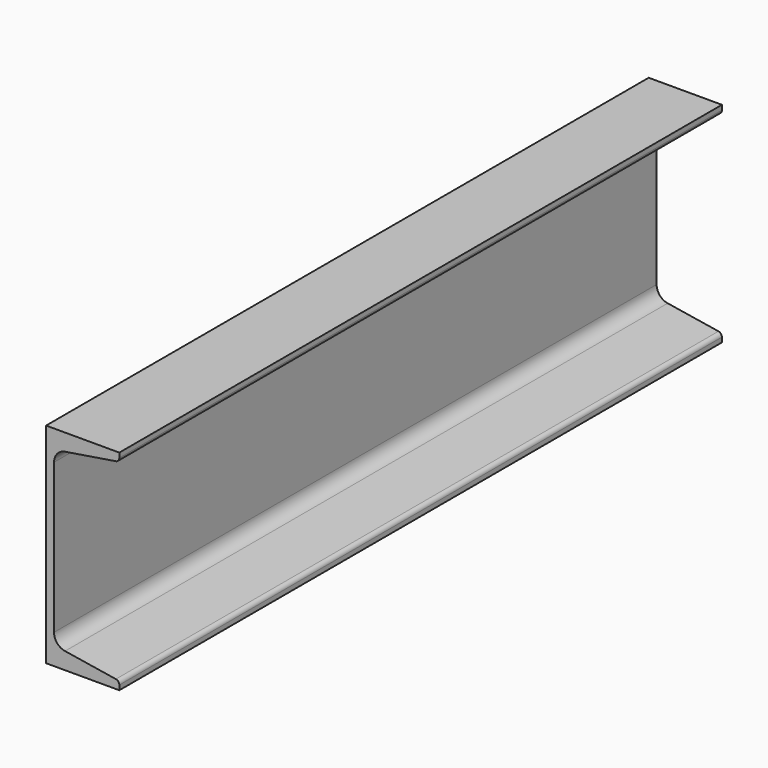
from build123d import *

# Parameters (mm, degrees)
F1_DEPTH = 457.2
F0_W     = 25.4
F0_H     = 49.170082
F0_H_2   = 8.8030812
F0_H_3   = 4.7118778
F0_W_2   = 31.496
F0_H_4   = 25.4
F0_W_3   = 6.5532254
F0_H_5   = 4.729226
F0_H_6   = 8.769477
F0_H_7   = 49.202594
F0_W_4   = 31.3436
F0_W_5   = 9.0424
F0_H_8   = 4.724908
F0_H_9   = 8.777859
F0_H_10  = 49.194466
F0_H_11  = 4.9884076
F0_H_12  = 10.7895644
F0_H_13  = 70.044056
F0_W_6   = 35.56
F0_W_7   = 8.1534
F0_H_14  = 90.86723
F0_H_15  = 12.7743204
F0_H_16  = 5.2920646
F0_W_8   = 39.6239238
F0_W_9   = 8.2550254
F0_H_17  = 7.9246984
F0_H_18  = 11.1253016
F0_H_19  = 88.9
F0_H_20  = 11.1252762
F0_H_21  = 7.9247238
F0_H_22  = 7.9249016
F0_H_23  = 12.7
F0_H_24  = 111.1501968
F0_W_10  = 46.8120476
F0_W_11  = 7.9756762
F0_H_25  = 111.1505778
F0_W_12  = 55.5499016
F0_W_13  = 7.8739238
F0_H_26  = 11.0997238
F0_H_27  = 9.525
F0_H_28  = 11.0996984
F0_H_29  = 111.1503746
F0_W_14  = 43.6878222
F0_W_15  = 11.0999016
F0_W_16  = 66.675
F0_W_17  = 8.0264508
F0_H_30  = 14.2746984
F0_H_31  = 98.4505778
F0_H_32  = 14.2747238
F0_W_18  = 80.2641016
F0_W_19  = 8.6358984
F0_H_33  = 20.6247238
F0_H_34  = 6.35
F0_H_35  = 20.6246984


# Not quite as in the source:
# - ends of sketch curves that miss each other by under 0.0002 mm in the source are joined


with BuildPart() as f1:
    # F0 (on Front) → F1 (new body)
    with BuildSketch(Plane.XZ):
        with BuildLine():
            Line((-601.1868342, 387.2012576), (-601.1868342, 311.0012576))
            Line((-601.1868342, 311.0012576), (-565.3728342, 311.0012576))
            Line((-565.3728342, 311.0012576), (-565.3728342, 313.5336122))
            ThreePointArc((-565.3728342, 313.5336122), (-565.9005539947, 314.9657928472), (-567.2313750211, 315.7131515187))
            Line((-567.2313750211, 315.7131515187), (-592.8587584, 319.8135336))
            ThreePointArc((-592.8587584, 319.8135336), (-595.7302015679, 321.4260723396), (-596.8688342, 324.5162166))
            Line((-596.8688342, 324.5162166), (-596.8688342, 373.6862986))
            ThreePointArc((-596.8688342, 373.6862986), (-595.7302015679, 376.7764428604), (-592.8587590083, 378.388985402))
            Line((-592.8587590083, 378.388985402), (-567.2313776, 382.4893798))
            ThreePointArc((-567.2313776, 382.4893798), (-565.9005539947, 383.2367223528), (-565.3728342, 384.668903))
            Line((-565.3728342, 384.668903), (-565.3728342, 387.2012576))
            Line((-565.3728342, 387.2012576), (-601.1868342, 387.2012576))
        make_face()
    extrude(amount=F1_DEPTH)


with BuildPart() as f1b:
    # F0 (on Front) → F1, piece 2 (new body)
    with BuildSketch(Plane.XZ):
        Polygon((-490.1583542, 311.0012576), (-458.6623542, 311.0012576), (-458.6623542, 336.4012576), (-490.1583542, 336.4012576), (-490.1583542, 315.3192576), align=None)
        Polygon((-494.4763542, 311.0012576), (-490.1583542, 311.0012576), (-490.1583542, 315.3192576), align=None)
        Polygon((-490.1583542, 315.3192576), (-490.1583542, 336.4012576), (-494.4763542, 336.4012576), (-494.4763542, 311.0012576), align=None)
    extrude(amount=F1_DEPTH)


with BuildPart() as f1c:
    # F0 (on Front) → F1, piece 3 (new body)
    with BuildSketch(Plane.XZ):
        with Locations((-369.8588742, 349.1012576)):
            Rectangle(F0_W, F0_H)
        with Locations((-369.8588742, 378.0878392)):
            Rectangle(F0_W, F0_H_2)
        with Locations((-369.8588742, 384.8453187)):
            Rectangle(F0_W, F0_H_3)
        Polygon((-357.1588742, 315.7131354), (-357.1588742, 324.5162166), (-382.5588742, 324.5162166), (-382.5588742, 315.7131354), (-377.8469964, 315.7131354), align=None)
        Polygon((-357.1588742, 311.0012576), (-357.1588742, 315.7131354), (-377.8469964, 315.7131354), (-382.5588742, 311.0012576), align=None)
        Polygon((-377.8469964, 315.7131354), (-382.5588742, 315.7131354), (-382.5588742, 311.0012576), align=None)
    extrude(amount=F1_DEPTH)


with BuildPart() as f1d:
    # F0 (on Front) → F1, piece 4 (new body)
    with BuildSketch(Plane.XZ):
        with BuildLine():
            Line((-282.0713942, 387.2012576), (-282.0713942, 311.0012576))
            Line((-282.0713942, 311.0012576), (-244.2253942, 311.0012576))
            Line((-244.2253942, 311.0012576), (-244.2253942, 313.542934))
            ThreePointArc((-244.2253942, 313.542934), (-244.755053678, 314.9803842916), (-246.0907679772, 315.7304974926))
            Line((-246.0907679772, 315.7304974926), (-271.5081184, 319.7972776))
            ThreePointArc((-271.5081184, 319.7972776), (-274.3795615679, 321.4098163396), (-275.5181942, 324.4999606))
            Line((-275.5181942, 324.4999606), (-275.5181942, 373.7025546))
            ThreePointArc((-275.5181942, 373.7025546), (-274.3795615679, 376.7926988604), (-271.5081190083, 378.405241402))
            Line((-271.5081190083, 378.405241402), (-246.0907702, 382.4720316))
            ThreePointArc((-246.0907702, 382.4720316), (-244.755053678, 383.2221309084), (-244.2253942, 384.6595812))
            Line((-244.2253942, 384.6595812), (-244.2253942, 387.2012576))
            Line((-244.2253942, 387.2012576), (-282.0713942, 387.2012576))
        make_face()
    extrude(amount=F1_DEPTH)


with BuildPart() as f1e:
    # F0 (on Front) → F1, piece 5 (new body)
    with BuildSketch(Plane.XZ):
        with Locations((-153.1612888, 323.7012576)):
            Rectangle(F0_W_2, F0_H_4)
        with Locations((-172.1859015, 323.7012576)):
            Rectangle(F0_W_3, F0_H_4)
    extrude(amount=F1_DEPTH)


with BuildPart() as f1f:
    # F0 (on Front) → F1, piece 6 (new body)
    with BuildSketch(Plane.XZ):
        with Locations((-49.7274342, 384.8366446)):
            Rectangle(F0_W, F0_H_5)
        with Locations((-49.7274342, 378.0872931)):
            Rectangle(F0_W, F0_H_6)
        with Locations((-49.7274342, 349.1012576)):
            Rectangle(F0_W, F0_H_7)
        Polygon((-37.0274342, 324.4999606), (-62.4274342, 324.4999606), (-62.4274342, 315.7304836), (-57.6982082, 315.7304836), (-37.0274342, 315.7304836), align=None)
        Polygon((-57.6982082, 315.7304836), (-62.4274342, 315.7304836), (-62.4274342, 311.0012576), align=None)
        Polygon((-57.6982082, 315.7304836), (-62.4274342, 311.0012576), (-37.0274342, 311.0012576), (-37.0274342, 315.7304836), align=None)
    extrude(amount=F1_DEPTH)


with BuildPart() as f1g:
    # F0 (on Front) → F1, piece 7 (new body)
    with BuildSketch(Plane.XZ):
        with BuildLine():
            Line((36.7900458, 387.2012576), (36.7900458, 311.0012576))
            Line((36.7900458, 311.0012576), (77.1760458, 311.0012576))
            Line((77.1760458, 311.0012576), (77.1760458, 313.5405972))
            ThreePointArc((77.1760458, 313.5405972), (76.6468679067, 314.9767339928), (75.3123701078, 315.7261562738))
            Line((75.3123701078, 315.7261562738), (49.8425216, 319.8013416))
            ThreePointArc((49.8425216, 319.8013416), (46.9710784321, 321.4138803396), (45.8324458, 324.5040246))
            Line((45.8324458, 324.5040246), (45.8324458, 373.6984906))
            ThreePointArc((45.8324458, 373.6984906), (46.9710784321, 376.7886348604), (49.8425209917, 378.401177402))
            Line((49.8425209917, 378.401177402), (75.3123716, 382.4763496))
            ThreePointArc((75.3123716, 382.4763496), (76.6468679067, 383.2257812072), (77.1760458, 384.661918))
            Line((77.1760458, 384.661918), (77.1760458, 387.2012576))
            Line((77.1760458, 387.2012576), (36.7900458, 387.2012576))
        make_face()
    extrude(amount=F1_DEPTH)


with BuildPart() as f1h:
    # F0 (on Front) → F1, piece 8 (new body)
    with BuildSketch(Plane.XZ):
        with Locations((168.2020258, 323.7012576)):
            Rectangle(F0_W_4, F0_H_4)
        with Locations((148.0090258, 323.7012576)):
            Rectangle(F0_W_5, F0_H_4)
    extrude(amount=F1_DEPTH)


with BuildPart() as f1i:
    # F0 (on Front) → F1, piece 9 (new body)
    with BuildSketch(Plane.XZ):
        with Locations((270.4040058, 384.8388036)):
            Rectangle(F0_W, F0_H_8)
        with Locations((270.4040058, 378.0874201)):
            Rectangle(F0_W, F0_H_9)
        with Locations((270.4040058, 349.1012576)):
            Rectangle(F0_W, F0_H_10)
        Polygon((283.1040058, 324.5040246), (257.7040058, 324.5040246), (257.7040058, 315.7261656), (262.4289138, 315.7261656), (283.1040058, 315.7261656), align=None)
        Polygon((262.4289138, 315.7261656), (257.7040058, 315.7261656), (257.7040058, 311.0012576), align=None)
        Polygon((262.4289138, 315.7261656), (257.7040058, 311.0012576), (283.1040058, 311.0012576), (283.1040058, 315.7261656), align=None)
    extrude(amount=F1_DEPTH)


with BuildPart() as f1j:
    # F0 (on Front) → F1, piece 10 (new body)
    with BuildSketch(Plane.XZ):
        with BuildLine():
            Line((356.9976858, 412.6012576), (356.9976858, 311.0012576))
            Line((356.9976858, 311.0012576), (397.2312858, 311.0012576))
            Line((397.2312858, 311.0012576), (397.2312858, 313.6822276))
            ThreePointArc((397.2312858, 313.6822276), (396.6725971949, 315.1984578291), (395.2636770123, 315.9896790272))
            Line((395.2636770123, 315.9896790272), (367.0180366, 320.5089856))
            ThreePointArc((367.0180366, 320.5089856), (363.1894572183, 322.6590436143), (361.6712858, 326.7792296))
            Line((361.6712858, 326.7792296), (361.6712858, 396.8232856))
            ThreePointArc((361.6712858, 396.8232856), (363.1894572183, 400.9434715857), (367.0180362116, 403.0935320276))
            Line((367.0180362116, 403.0935320276), (395.2636748, 407.61285))
            ThreePointArc((395.2636748, 407.61285), (396.6725971949, 408.4040573709), (397.2312858, 409.9202876))
            Line((397.2312858, 409.9202876), (397.2312858, 412.6012576))
            Line((397.2312858, 412.6012576), (356.9976858, 412.6012576))
        make_face()
    extrude(amount=F1_DEPTH)


with BuildPart() as f1k:
    # F0 (on Front) → F1, piece 11 (new body)
    with BuildSketch(Plane.XZ):
        Polygon((468.3817658, 336.4012576), (463.7081658, 336.4012576), (463.7081658, 311.0012576), (468.3817658, 315.6748576), align=None)
        Polygon((503.9417658, 336.4012576), (468.3817658, 336.4012576), (468.3817658, 315.6748576), (468.3817658, 311.0012576), (503.9417658, 311.0012576), align=None)
        Polygon((468.3817658, 315.6748576), (463.7081658, 311.0012576), (468.3817658, 311.0012576), align=None)
    extrude(amount=F1_DEPTH)


with BuildPart() as f1l:
    # F0 (on Front) → F1, piece 12 (new body)
    with BuildSketch(Plane.XZ):
        with Locations((590.5354458, 410.1070538)):
            Rectangle(F0_W, F0_H_11)
        with Locations((590.5354458, 402.2180678)):
            Rectangle(F0_W, F0_H_12)
        with Locations((590.5354458, 361.8012576)):
            Rectangle(F0_W, F0_H_13)
        Polygon((603.2354458, 315.9896652), (603.2354458, 326.7792296), (577.8354458, 326.7792296), (577.8354458, 315.9896652), (582.8238534, 315.9896652), align=None)
        Polygon((603.2354458, 311.0012576), (603.2354458, 315.9896652), (582.8238534, 315.9896652), (577.8354458, 311.0012576), align=None)
        Polygon((577.8354458, 311.0012576), (582.8238534, 315.9896652), (577.8354458, 315.9896652), align=None)
    extrude(amount=F1_DEPTH)


with BuildPart() as f1m:
    # F0 (on Front) → F1, piece 13 (new body)
    with BuildSketch(Plane.XZ):
        with BuildLine():
            ThreePointArc((-591.6363837884, 89.6092671724), (-595.4649627817, 91.7593276143), (-596.9831342, 95.8795136))
            Line((-596.9831342, 95.8795136), (-596.9831342, 165.9235696))
            ThreePointArc((-596.9831342, 165.9235696), (-595.4649627817, 170.0437555857), (-591.6363837884, 172.1938160276))
            Line((-591.6363837884, 172.1938160276), (-563.3907452, 176.713134))
            ThreePointArc((-563.3907452, 176.713134), (-561.9818228051, 177.5043413709), (-561.4231342, 179.0205716))
            Line((-561.4231342, 179.0205716), (-561.4231342, 181.7015416))
            Line((-561.4231342, 181.7015416), (-605.1365342, 181.7015416))
            Line((-605.1365342, 181.7015416), (-605.1365342, 80.1015416))
            Line((-605.1365342, 80.1015416), (-561.4231342, 80.1015416))
            Line((-561.4231342, 80.1015416), (-561.4231342, 82.7825116))
            ThreePointArc((-561.4231342, 82.7825116), (-561.9818228051, 84.2987418291), (-563.3907429877, 85.0899630272))
            Line((-563.3907429877, 85.0899630272), (-591.6363837884, 89.6092671724))
        make_face()
    extrude(amount=F1_DEPTH)


with BuildPart() as f1n:
    # F0 (on Front) → F1, piece 14 (new body)
    with BuildSketch(Plane.XZ):
        with Locations((-472.5053542, 92.8015416)):
            Rectangle(F0_W_6, F0_H_4)
        with Locations((-494.3620542, 92.8015416)):
            Rectangle(F0_W_7, F0_H_4)
    extrude(amount=F1_DEPTH)


with BuildPart() as f1o:
    # F0 (on Front) → F1, piece 15 (new body)
    with BuildSketch(Plane.XZ):
        Polygon((-382.5588742, 80.1015416), (-357.1588742, 80.1015416), (-357.1588742, 85.0899492), (-377.5704666, 85.0899492), align=None)
        Polygon((-382.5588742, 85.0899492), (-382.5588742, 80.1015416), (-377.5704666, 85.0899492), align=None)
        Polygon((-377.5704666, 85.0899492), (-357.1588742, 85.0899492), (-357.1588742, 95.8795136), (-382.5588742, 95.8795136), (-382.5588742, 85.0899492), align=None)
        with Locations((-369.8588742, 130.9015416)):
            Rectangle(F0_W, F0_H_13)
        with Locations((-369.8588742, 171.3183518)):
            Rectangle(F0_W, F0_H_12)
        with Locations((-369.8588742, 179.2073378)):
            Rectangle(F0_W, F0_H_11)
    extrude(amount=F1_DEPTH)


with BuildPart() as f1p:
    # F0 (on Front) → F1, piece 16 (new body)
    with BuildSketch(Plane.XZ):
        with BuildLine():
            Line((-285.3733942, 207.1015416), (-285.3733942, 80.1015416))
            Line((-285.3733942, 80.1015416), (-240.9233942, 80.1015416))
            Line((-240.9233942, 80.1015416), (-240.9233942, 82.9457066))
            ThreePointArc((-240.9233942, 82.9457066), (-241.5160882904, 84.5542271722), (-243.0107654656, 85.3936107901))
            Line((-243.0107654656, 85.3936107901), (-273.863943, 90.3301216))
            ThreePointArc((-273.863943, 90.3301216), (-278.6496758587, 93.0176893467), (-280.5473942, 98.1679266))
            Line((-280.5473942, 98.1679266), (-280.5473942, 189.0351566))
            ThreePointArc((-280.5473942, 189.0351566), (-278.6496758587, 194.1853938533), (-273.8639438025, 196.8729666158))
            Line((-273.8639438025, 196.8729666158), (-243.0107662, 201.809477))
            ThreePointArc((-243.0107662, 201.809477), (-241.5160882904, 202.6488560278), (-240.9233942, 204.2573766))
            Line((-240.9233942, 204.2573766), (-240.9233942, 207.1015416))
            Line((-240.9233942, 207.1015416), (-285.3733942, 207.1015416))
        make_face()
    extrude(amount=F1_DEPTH)


with BuildPart() as f1q:
    # F0 (on Front) → F1, piece 17 (new body)
    with BuildSketch(Plane.XZ):
        Polygon((-173.8369142, 80.1015416), (-134.2129142, 80.1015416), (-134.2129142, 105.5015416), (-173.8369142, 105.5015416), (-173.8369142, 84.9275416), align=None)
        Polygon((-178.6629142, 80.1015416), (-173.8369142, 80.1015416), (-173.8369142, 84.9275416), align=None)
        Polygon((-173.8369142, 84.9275416), (-173.8369142, 105.5015416), (-178.6629142, 105.5015416), (-178.6629142, 80.1015416), align=None)
    extrude(amount=F1_DEPTH)


with BuildPart() as f1r:
    # F0 (on Front) → F1, piece 18 (new body)
    with BuildSketch(Plane.XZ):
        Polygon((-62.4274342, 80.1015416), (-37.0274342, 80.1015416), (-37.0274342, 85.3936062), (-57.1353696, 85.3936062), align=None)
        Polygon((-57.1353696, 85.3936062), (-37.0274342, 85.3936062), (-37.0274342, 98.1679266), (-62.4274342, 98.1679266), (-62.4274342, 85.3936062), align=None)
        Polygon((-62.4274342, 85.3936062), (-62.4274342, 80.1015416), (-57.1353696, 85.3936062), align=None)
        with Locations((-49.7274342, 143.6015416)):
            Rectangle(F0_W, F0_H_14)
        with Locations((-49.7274342, 195.4223168)):
            Rectangle(F0_W, F0_H_15)
        with Locations((-49.7274342, 204.4555093)):
            Rectangle(F0_W, F0_H_16)
    extrude(amount=F1_DEPTH)


with BuildPart() as f1s:
    # F0 (on Front) → F1, piece 19 (new body)
    with BuildSketch(Plane.XZ):
        with BuildLine():
            ThreePointArc((47.9819961975, 90.3301165842), (43.1962641413, 93.0176893467), (41.2985458, 98.1679266))
            Line((41.2985458, 98.1679266), (41.2985458, 189.0351566))
            ThreePointArc((41.2985458, 189.0351566), (43.1962641413, 194.1853938533), (47.9819961975, 196.8729666158))
            Line((47.9819961975, 196.8729666158), (78.8351738, 201.809477))
            ThreePointArc((78.8351738, 201.809477), (80.3298517096, 202.6488560278), (80.9225458, 204.2573766))
            Line((80.9225458, 204.2573766), (80.9225458, 207.1015416))
            Line((80.9225458, 207.1015416), (33.0435458, 207.1015416))
            Line((33.0435458, 207.1015416), (33.0435458, 80.1015416))
            Line((33.0435458, 80.1015416), (80.9225458, 80.1015416))
            Line((80.9225458, 80.1015416), (80.9225458, 82.9457066))
            ThreePointArc((80.9225458, 82.9457066), (80.3298517096, 84.5542271722), (78.8351745344, 85.3936107901))
            Line((78.8351745344, 85.3936107901), (47.9819961975, 90.3301165842))
        make_face()
    extrude(amount=F1_DEPTH)


with BuildPart() as f1t:
    # F0 (on Front) → F1, piece 20 (new body)
    with BuildSketch(Plane.XZ):
        with Locations((167.8083131, 92.8015416)):
            Rectangle(F0_W_8, F0_H_4)
        with Locations((143.8688385, 92.8015416)):
            Rectangle(F0_W_9, F0_H_4)
    extrude(amount=F1_DEPTH)


with BuildPart() as f1u:
    # F0 (on Front) → F1, piece 21 (new body)
    with BuildSketch(Plane.XZ):
        with Locations((270.4040058, 84.0638908)):
            Rectangle(F0_W, F0_H_17)
        with Locations((270.4040058, 93.5888908)):
            Rectangle(F0_W, F0_H_18)
        with Locations((270.4040058, 143.6015416)):
            Rectangle(F0_W, F0_H_19)
        with Locations((270.4040058, 193.6141797)):
            Rectangle(F0_W, F0_H_20)
        with Locations((270.4040058, 203.1391797)):
            Rectangle(F0_W, F0_H_21)
    extrude(amount=F1_DEPTH)


with BuildPart() as f1v:
    # F0 (on Front) → F1, piece 22 (new body)
    with BuildSketch(Plane.XZ):
        with BuildLine():
            ThreePointArc((365.8306401459, 91.025565362), (360.0877523662, 94.2506495524), (357.8104858, 100.4309396))
            Line((357.8104858, 100.4309396), (357.8104858, 212.1721436))
            ThreePointArc((357.8104858, 212.1721436), (360.0877523662, 218.3524336476), (365.8306401459, 221.577517838))
            Line((365.8306401459, 221.577517838), (399.3020462, 226.9329472))
            ThreePointArc((399.3020462, 226.9329472), (400.8748228991, 227.816191046), (401.4984858, 229.5087612))
            Line((401.4984858, 229.5087612), (401.4984858, 232.5015416))
            Line((401.4984858, 232.5015416), (352.7304858, 232.5015416))
            Line((352.7304858, 232.5015416), (352.7304858, 80.1015416))
            Line((352.7304858, 80.1015416), (401.4984858, 80.1015416))
            Line((401.4984858, 80.1015416), (401.4984858, 83.094322))
            ThreePointArc((401.4984858, 83.094322), (400.8748228991, 84.786892154), (399.3020465678, 85.6701382986))
            Line((399.3020465678, 85.6701382986), (365.8306401459, 91.025565362))
        make_face()
    extrude(amount=F1_DEPTH)


with BuildPart() as f1w:
    # F0 (on Front) → F1, piece 23 (new body)
    with BuildSketch(Plane.XZ):
        Polygon((464.5209912, 80.1015416), (508.208915, 80.1015416), (508.208915, 105.5015416), (464.5209912, 105.5015416), (464.5209912, 85.181567), align=None)
        Polygon((459.4409658, 80.1015416), (464.5209912, 80.1015416), (464.5209912, 85.181567), align=None)
        Polygon((464.5209912, 85.181567), (464.5209912, 105.5015416), (459.4409658, 105.5015416), (459.4409658, 80.1015416), align=None)
    extrude(amount=F1_DEPTH)


with BuildPart() as f1x:
    # F0 (on Front) → F1, piece 24 (new body)
    with BuildSketch(Plane.XZ):
        with Locations((590.5354458, 228.5390908)):
            Rectangle(F0_W, F0_H_22)
        with Locations((590.5354458, 218.22664)):
            Rectangle(F0_W, F0_H_23)
        with Locations((590.5354458, 156.3015416)):
            Rectangle(F0_W, F0_H_24)
        with Locations((590.5354458, 94.3764432)):
            Rectangle(F0_W, F0_H_23)
        with Locations((590.5354458, 84.0639924)):
            Rectangle(F0_W, F0_H_22)
    extrude(amount=F1_DEPTH)


with BuildPart() as f1y:
    # F0 (on Front) → F1, piece 25 (new body)
    with BuildSketch(Plane.XZ):
        with BuildLine():
            Line((-609.1116342, 1.6018256), (-609.1116342, -150.7981744))
            Line((-609.1116342, -150.7981744), (-557.4480342, -150.7981744))
            Line((-557.4480342, -150.7981744), (-557.4480342, -147.805394))
            ThreePointArc((-557.4480342, -147.805394), (-558.0716971009, -146.112823846), (-559.6444734322, -145.2295777014))
            Line((-559.6444734322, -145.2295777014), (-593.1158826, -139.8741678))
            ThreePointArc((-593.1158826, -139.8741678), (-598.8587676338, -136.6490664476), (-601.1360342, -130.4687764))
            Line((-601.1360342, -130.4687764), (-601.1360342, -18.7275724))
            ThreePointArc((-601.1360342, -18.7275724), (-598.8587676338, -12.5472823524), (-593.1158798541, -9.322198162))
            Line((-593.1158798541, -9.322198162), (-559.6444738, -3.9667688))
            ThreePointArc((-559.6444738, -3.9667688), (-558.0716971009, -3.083524954), (-557.4480342, -1.3909548))
            Line((-557.4480342, -1.3909548), (-557.4480342, 1.6018256))
            Line((-557.4480342, 1.6018256), (-609.1116342, 1.6018256))
        make_face()
    extrude(amount=F1_DEPTH)


with BuildPart() as f1z:
    # F0 (on Front) → F1, piece 26 (new body)
    with BuildSketch(Plane.XZ):
        with Locations((-472.5942542, -138.0981744)):
            Rectangle(F0_W_10, F0_H_4)
        with Locations((-499.9881161, -138.0981744)):
            Rectangle(F0_W_11, F0_H_4)
    extrude(amount=F1_DEPTH)


with BuildPart() as f1ba:
    # F0 (on Front) → F1, piece 27 (new body)
    with BuildSketch(Plane.XZ):
        with Locations((-369.8588742, -146.8358252)):
            Rectangle(F0_W, F0_H_17)
        with Locations((-369.8588742, -136.523476)):
            Rectangle(F0_W, F0_H_23)
        with Locations((-369.8588742, -74.5981871)):
            Rectangle(F0_W, F0_H_25)
        with Locations((-369.8588742, -12.6728982)):
            Rectangle(F0_W, F0_H_23)
        with Locations((-369.8588742, -2.3605363)):
            Rectangle(F0_W, F0_H_21)
    extrude(amount=F1_DEPTH)


with BuildPart() as f1bb:
    # F0 (on Front) → F1, piece 28 (new body)
    with BuildSketch(Plane.XZ):
        with BuildLine():
            Line((-294.8602942, 1.6018256), (-294.8602942, -150.7981744))
            Line((-294.8602942, -150.7981744), (-231.4364942, -150.7981744))
            Line((-231.4364942, -150.7981744), (-231.4364942, -147.883499))
            ThreePointArc((-231.4364942, -147.883499), (-232.043887476, -146.2350911736), (-233.5756320118, -145.3748972241))
            Line((-233.5756320118, -145.3748972241), (-278.9661426, -138.1124238))
            ThreePointArc((-278.9661426, -138.1124238), (-284.7090276338, -134.8873224476), (-286.9862942, -128.7070324))
            Line((-286.9862942, -128.7070324), (-286.9862942, -20.4893164))
            ThreePointArc((-286.9862942, -20.4893164), (-284.7090276338, -14.3090263524), (-278.9661398541, -11.083942162))
            Line((-278.9661398541, -11.083942162), (-233.5756314, -3.8214554))
            ThreePointArc((-233.5756314, -3.8214554), (-232.043887476, -2.9612576264), (-231.4364942, -1.3128498))
            Line((-231.4364942, -1.3128498), (-231.4364942, 1.6018256))
            Line((-231.4364942, 1.6018256), (-294.8602942, 1.6018256))
        make_face()
    extrude(amount=F1_DEPTH)


with BuildPart() as f1bc:
    # F0 (on Front) → F1, piece 29 (new body)
    with BuildSketch(Plane.XZ):
        with Locations((-152.5009396, -138.0981744)):
            Rectangle(F0_W_12, F0_H_4)
        with Locations((-184.2128523, -138.0981744)):
            Rectangle(F0_W_13, F0_H_4)
    extrude(amount=F1_DEPTH)


with BuildPart() as f1bd:
    # F0 (on Front) → F1, piece 30 (new body)
    with BuildSketch(Plane.XZ):
        with Locations((-49.7274342, -13.4730363)):
            Rectangle(F0_W, F0_H_26)
        with Locations((-49.7274342, -74.5981871)):
            Rectangle(F0_W, F0_H_25)
        with Locations((-49.7274342, -3.1606744)):
            Rectangle(F0_W, F0_H_27)
        with Locations((-49.7274342, -135.7233252)):
            Rectangle(F0_W, F0_H_28)
        with Locations((-49.7274342, -146.0356744)):
            Rectangle(F0_W, F0_H_27)
    extrude(amount=F1_DEPTH)


with BuildPart() as f1be:
    # F0 (on Front) → F1, piece 31 (new body)
    with BuildSketch(Plane.XZ):
        with BuildLine():
            Line((29.5891458, 1.6018256), (29.5891458, -150.7981744))
            Line((29.5891458, -150.7981744), (84.3769458, -150.7981744))
            Line((84.3769458, -150.7981744), (84.3769458, -147.805394))
            ThreePointArc((84.3769458, -147.805394), (83.7532828991, -146.112823846), (82.1805065678, -145.2295777014))
            Line((82.1805065678, -145.2295777014), (48.7090974, -139.8741678))
            ThreePointArc((48.7090974, -139.8741678), (42.9662123662, -136.6490664476), (40.6889458, -130.4687764))
            Line((40.6889458, -130.4687764), (40.6889458, -18.7275724))
            ThreePointArc((40.6889458, -18.7275724), (42.9662123662, -12.5472823524), (48.7091001459, -9.322198162))
            Line((48.7091001459, -9.322198162), (82.1805062, -3.9667688))
            ThreePointArc((82.1805062, -3.9667688), (83.7532828991, -3.083524954), (84.3769458, -1.3909548))
            Line((84.3769458, -1.3909548), (84.3769458, 1.6018256))
            Line((84.3769458, 1.6018256), (29.5891458, 1.6018256))
        make_face()
    extrude(amount=F1_DEPTH)


with BuildPart() as f1bf:
    # F0 (on Front) → F1, piece 32 (new body)
    with BuildSketch(Plane.XZ):
        with Locations((163.6935258, -74.5982633)):
            Rectangle(F0_W, F0_H_29)
        with Locations((163.6935258, -136.5234506)):
            Rectangle(F0_W, F0_H_23)
        with Locations((163.6935258, -12.673076)):
            Rectangle(F0_W, F0_H_23)
        with Locations((163.6935258, -146.8358125)):
            Rectangle(F0_W, F0_H_21)
        with Locations((163.6935258, -2.3606252)):
            Rectangle(F0_W, F0_H_22)
    extrude(amount=F1_DEPTH)


with BuildPart() as f1bg:
    # F0 (on Front) → F1, piece 33 (new body)
    with BuildSketch(Plane.XZ):
        with Locations((275.9412185, -138.0981744)):
            Rectangle(F0_W_14, F0_H_4)
        with Locations((248.5473566, -138.0981744)):
            Rectangle(F0_W_15, F0_H_4)
    extrude(amount=F1_DEPTH)


with BuildPart() as f1bh:
    # F0 (on Front) → F1, piece 34 (new body)
    with BuildSketch(Plane.XZ):
        with BuildLine():
            Line((339.7637858, 1.6018256), (339.7637858, -150.7981744))
            Line((339.7637858, -150.7981744), (414.4651858, -150.7981744))
            Line((414.4651858, -150.7981744), (414.4651858, -146.9369934))
            ThreePointArc((414.4651858, -146.9369934), (413.6605551761, -144.7532950948), (411.6314087753, -143.6137629043))
            Line((411.6314087753, -143.6137629043), (355.8103374, -134.6824078))
            ThreePointArc((355.8103374, -134.6824078), (350.0674523662, -131.4573064476), (347.7901858, -125.2770164))
            Line((347.7901858, -125.2770164), (347.7901858, -23.9193324))
            ThreePointArc((347.7901858, -23.9193324), (350.0674523662, -17.7390423524), (355.8103401459, -14.513958162))
            Line((355.8103401459, -14.513958162), (411.6314094, -5.5825898))
            ThreePointArc((411.6314094, -5.5825898), (413.6605551761, -4.4430537052), (414.4651858, -2.2593554))
            Line((414.4651858, -2.2593554), (414.4651858, 1.6018256))
            Line((414.4651858, 1.6018256), (339.7637858, 1.6018256))
        make_face()
    extrude(amount=F1_DEPTH)


with BuildPart() as f1bi:
    # F0 (on Front) → F1, piece 35 (new body)
    with BuildSketch(Plane.XZ):
        with Locations((487.8382166, -138.0981744)):
            Rectangle(F0_W_16, F0_H_4)
        with Locations((450.4874912, -138.0981744)):
            Rectangle(F0_W_17, F0_H_4)
    extrude(amount=F1_DEPTH)


with BuildPart() as f1bj:
    # F0 (on Front) → F1, piece 36 (new body)
    with BuildSketch(Plane.XZ):
        with Locations((590.5354458, -144.4481744)):
            Rectangle(F0_W, F0_H_23)
        with Locations((590.5354458, -130.9608252)):
            Rectangle(F0_W, F0_H_30)
        with Locations((590.5354458, -74.5981871)):
            Rectangle(F0_W, F0_H_31)
        with Locations((590.5354458, -18.2355363)):
            Rectangle(F0_W, F0_H_32)
        with Locations((590.5354458, -4.7481744)):
            Rectangle(F0_W, F0_H_23)
    extrude(amount=F1_DEPTH)


with BuildPart() as f1bk:
    # F0 (on Front) → F1, piece 37 (new body)
    with BuildSketch(Plane.XZ):
        with BuildLine():
            Line((-621.3798342, -229.2978904), (-621.3798342, -381.6978904))
            Line((-621.3798342, -381.6978904), (-545.1798342, -381.6978904))
            Line((-545.1798342, -381.6978904), (-545.1798342, -377.8367094))
            ThreePointArc((-545.1798342, -377.8367094), (-545.9844648239, -375.6530110948), (-548.0136112247, -374.5134789043))
            Line((-548.0136112247, -374.5134789043), (-603.8346826, -365.5821238))
            ThreePointArc((-603.8346826, -365.5821238), (-609.5775676338, -362.3570224476), (-611.8548342, -356.1767324))
            Line((-611.8548342, -356.1767324), (-611.8548342, -254.8190484))
            ThreePointArc((-611.8548342, -254.8190484), (-609.5775676338, -248.6387583524), (-603.8346798541, -245.413674162))
            Line((-603.8346798541, -245.413674162), (-548.0136106, -236.4823058))
            ThreePointArc((-548.0136106, -236.4823058), (-545.9844648239, -235.3427697052), (-545.1798342, -233.1590714))
            Line((-545.1798342, -233.1590714), (-545.1798342, -229.2978904))
            Line((-545.1798342, -229.2978904), (-621.3798342, -229.2978904))
        make_face()
    extrude(amount=F1_DEPTH)


with BuildPart() as f1bl:
    # F0 (on Front) → F1, piece 38 (new body)
    with BuildSketch(Plane.XZ):
        with Locations((-472.264105, -368.9978904)):
            Rectangle(F0_W_18, F0_H_4)
        with Locations((-516.714105, -368.9978904)):
            Rectangle(F0_W_19, F0_H_4)
    extrude(amount=F1_DEPTH)


with BuildPart() as f1bm:
    # F0 (on Front) → F1, piece 39 (new body)
    with BuildSketch(Plane.XZ):
        with Locations((-369.8588742, -245.9602523)):
            Rectangle(F0_W, F0_H_33)
        with Locations((-369.8588742, -305.4979031)):
            Rectangle(F0_W, F0_H_31)
        with Locations((-369.8588742, -232.4728904)):
            Rectangle(F0_W, F0_H_34)
        with Locations((-369.8588742, -365.0355412)):
            Rectangle(F0_W, F0_H_35)
        with Locations((-369.8588742, -378.5228904)):
            Rectangle(F0_W, F0_H_34)
    extrude(amount=F1_DEPTH)


solid = f1p.part
